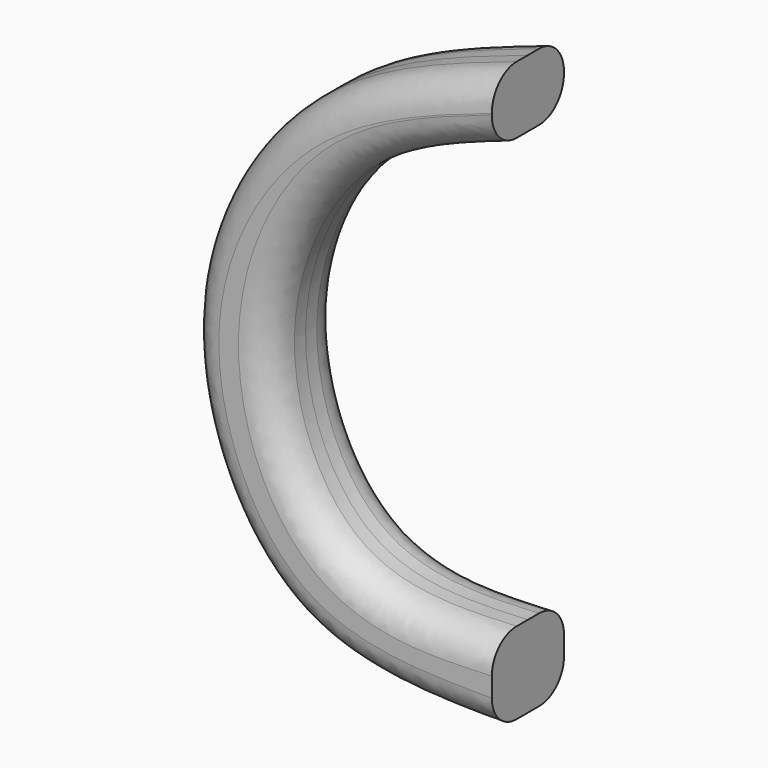
from build123d import *

# Parameters (mm, degrees)
F1_DEPTH = 4.445
F2_R     = 3.0660512242


with BuildPart() as f1:
    # F0 (on Front) → F1 (new body, symmetric)
    with BuildSketch(Plane.XZ):
        with BuildLine():
            add(Edge.make_bspline(
                [(0, 24.8093027622), (-5.3070638963, 22.9463474844), (-16.243352269, 19.1073478904), (-24.6673743675, 0.3717245375), (-16.8420720167, -18.329353742), (-5.5262778619, -17.8213493893), (0, -17.5732560456)],
                knots=[0, 0, 0, 0, 0.2483271457, 0.5117287692, 0.7615436923, 1, 1, 1, 1], degree=3))
            Line((0, 24.8093027622), (0, 31.4279086888))
            add(Edge.make_bspline(
                [(0, 31.4279086888), (-7.0194354851, 29.0510668461), (-21.3918948766, 24.1844272229), (-34.0931470298, 0.5079335618), (-22.5379858632, -25.4600909734), (-7.3456795521, -25.578855667), (0, -25.6362799555)],
                knots=[0, 0, 0, 0, 0.2465113826, 0.5047378588, 0.7605342527, 1, 1, 1, 1], degree=3))
            Line((0, -25.6362799555), (0, -17.5732560456))
        make_face()
    extrude(amount=F1_DEPTH, both=True)

    # F2
    f2_edges = [f1.edges().sort_by_distance(p)[0] for p in [
        (-29.957392, -4.445, 0.657837),
        (-29.957392, 4.445, 0.657837),
        (-21.865566, 4.445, 1.442691),
        (-21.865566, -4.445, 1.442691),
    ]]
    fillet(f2_edges, radius=F2_R)


solid = f1.part
